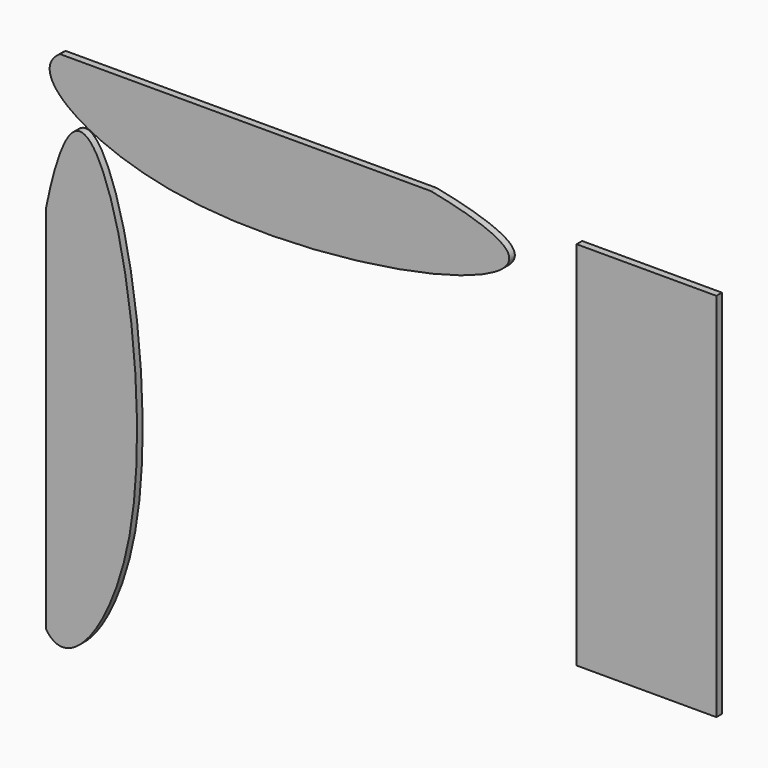
from build123d import *

# Parameters (mm, degrees)
F0_W     = 63.5
F0_H     = 168.5544
F1_DEPTH = 3.175


# Not quite as in the source:
# - a length typed as a fraction of an inch, garbled in the dataset ("3 / 203.2 mm" for 3/8 in), is restored
# - a feature names something its author has since deleted; it is built from what else it names


with BuildPart() as f1:
    # F0 (on Front) → F1 (new body)
    with BuildSketch(Plane.XZ):
        with Locations((120.65, 68.1228)):
            Rectangle(F0_W, F0_H)
    extrude(amount=F1_DEPTH)


with BuildPart() as f1b:
    # F0 (on Front) → F1, piece 2 (new body)
    with BuildSketch(Plane.XZ):
        with BuildLine():
            add(Edge.make_bspline(
                [(-145.852143538, 152.1171118736), (-161.6387986112, 141.6337447271), (-95.7451417453, 89.5280224527), (98.5891023928, 129.2431554146), (40.7846440978, 148.5452015878), (22.7073728104, 152.1171118736)],
                knots=[0, 0, 0, 0, 0.2298618019, 0.5884097433, 0.6935771532, 0.6935771532, 0.6935771532, 0.6935771532], degree=3))
            Line((22.7073728104, 152.1171118736), (-145.852143538, 152.1171118736))
        make_face()
    extrude(amount=F1_DEPTH)


with BuildPart() as f1c:
    # F0 (on Front) → F1, piece 3 (new body)
    with BuildSketch(Plane.XZ):
        with BuildLine():
            Line((-152.1824385643, 88.5141490955), (-152.1824385643, -80.0453672528))
            add(Edge.make_bspline(
                [(-152.1824385643, -80.0453672528), (-141.6990714177, -95.832022326), (-89.5933491434, -29.9383654601), (-129.3084821052, 164.395878678), (-148.6105282784, 106.5914203829), (-152.1824385643, 88.5141490955)],
                knots=[0, 0, 0, 0, 0.2298618019, 0.5884097433, 0.6935771532, 0.6935771532, 0.6935771532, 0.6935771532], degree=3))
        make_face()
    extrude(amount=F1_DEPTH)


solid = Compound([f1.part, f1b.part, f1c.part])
